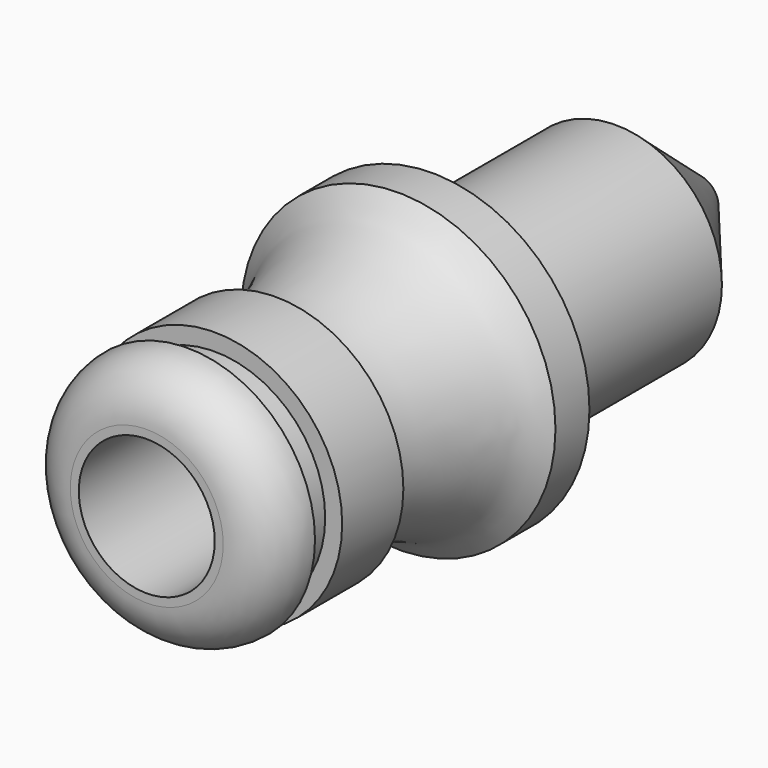
from build123d import *

# Parameters (mm, degrees)
F0_W = 2.25
F0_H = 10.4924628735
F2_R = 2.99999


# Not quite as in the source:
# - a fillet or chamfer is up to 0.001 mm smaller than in the source, because OpenCascade refuses the exact size


with BuildPart() as f1:
    # F0 (on Top) → F1 (revolve)
    with BuildSketch(Plane.XY):
        with BuildLine():
            Line((4, 10), (4, 0))
            Line((4, 0), (7.5, 0))
            Line((7.5, 0), (7.5, 3))
            Line((7.5, 3), (6.5, 3))
            Line((6.5, 3), (6.5, 5))
            Line((6.5, 5), (7.5, 5))
            Line((7.5, 5), (7.5, 9.5))
            Line((7.5, 9.5), (6.1, 9.5))
            add(Edge.make_bspline(
                [(6.1, 9.5), (6.0997806749, 9.542689319), (6.0997821122, 9.585377965), (6.1, 9.6280611679)],
                knots=[0, 0, 0, 0, 0.0093487262, 0.0093487262, 0.0093487262, 0.0093487262], degree=3))
            add(Edge.make_bspline(
                [(6.1, 9.6280611679), (6.1147869444, 12.5247545063), (7.6944598018, 17.0085980566), (8.4188714562, 17.7962221352), (9.25, 18.5)],
                knots=[0.0093487262, 0.0093487262, 0.0093487262, 0.0093487262, 0.6437995433, 1, 1, 1, 1], degree=3))
            Line((9.25, 18.5), (9.25, 21))
            Line((9.25, 21), (6.25, 21))
            Line((6.25, 21), (6.25, 24))
            Line((6.25, 24), (4, 24))
            Line((4, 24), (4, 10))
        make_face()
        with Locations((5.125, 29.2462314367)):
            Rectangle(F0_W, F0_H)
        Polygon((1.25, 37.7924628735), (4, 34.4924628735), (6.25, 34.4924628735), (1.25, 40.4924628735), align=None)
        with BuildLine():
            Line((6.1, 9.5), (6.1, 9.6280611679))
            add(Edge.make_bspline(
                [(6.1, 9.5), (6.0997806749, 9.542689319), (6.0997821122, 9.585377965), (6.1, 9.6280611679)],
                knots=[0, 0, 0, 0, 0.0093487262, 0.0093487262, 0.0093487262, 0.0093487262], degree=3))
        make_face()
    revolve(axis=Axis((0, 14.3348099664, 0), (0, 1, 0)))

    # F2 (radius 3 in the source; OpenCascade refuses exactly that, so slightly less here)
    f2_edges = [f1.edges().sort_by_distance(p)[0] for p in [
        (-7.5, 0, 0),
    ]]
    fillet(f2_edges, radius=F2_R)


solid = f1.part
